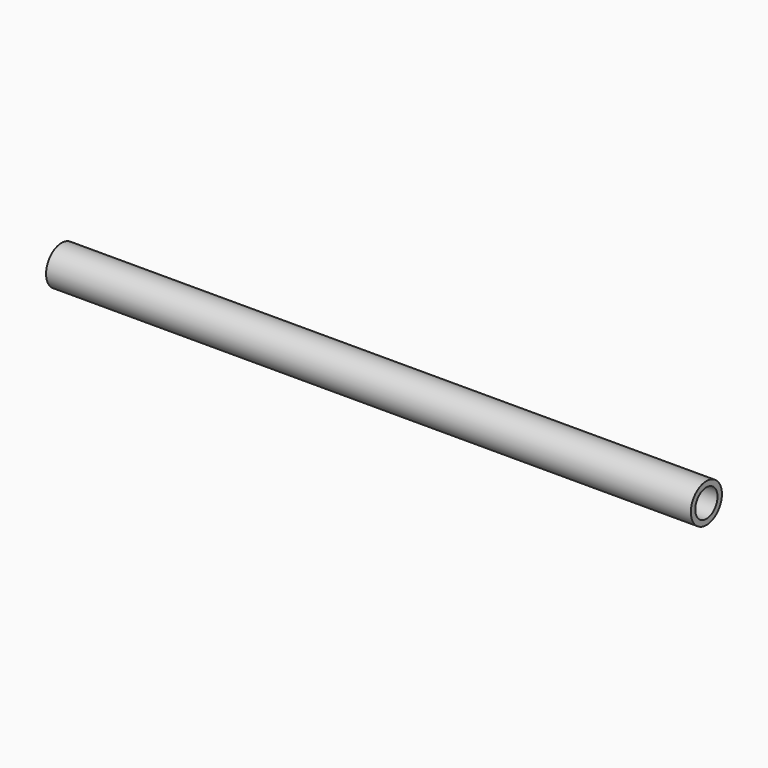
from build123d import *

# Parameters (mm, degrees)
F0_R     = 10.6426
F0_R_2   = 7.62
F1_DEPTH = 176.7205


# Not quite as in the source:
# - a length typed as a fraction of an inch, garbled in the dataset ("3 / 203.2 mm" for 3/8 in), is restored


with BuildPart() as f1:
    # F0 (on Right) → F1 (new body, symmetric)
    with BuildSketch(Plane.YZ):
        Circle(F0_R)
        Circle(F0_R_2, mode=Mode.SUBTRACT)
    extrude(amount=F1_DEPTH, both=True)


solid = f1.part
